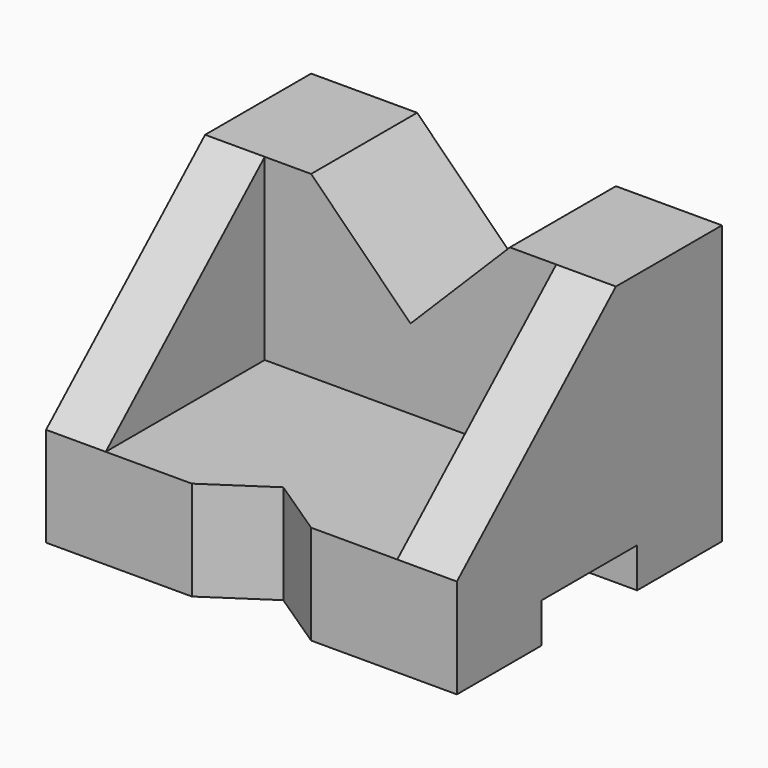
from build123d import *

# Parameters (mm, degrees)
F0_W      = 62
F0_H      = 15
F1_DEPTH  = 50
F3_DEPTH  = 20
F7_DEPTH  = 62
F8_DEPTH  = 9
F10_DEPTH = 25


# Not quite as in the source:
# - a pattern or mirror of a feature is missing from the dataset's text; its kind, count and spacing are read off the source's solid


with BuildPart() as f1:
    # F0 (on Front) → F1 (new body)
    with BuildSketch(Plane.XZ):
        with Locations((0, 7.5)):
            Rectangle(F0_W, F0_H)
    extrude(amount=F1_DEPTH)

    # F2 (on face) → F3 (join)
    with BuildSketch(Plane(origin=(0, 0, 0), x_dir=(-1, 0, 0), z_dir=(0, 1, 0))):
        Polygon((-31, 15), (31, 15), (31, 42), (15, 42), (0, 27), (-15, 42), (-31, 42), align=None)
    extrude(amount=-F3_DEPTH)

    # F5 (on face) → F7 (cut)
    with BuildSketch(Plane(origin=(-31, 0, 0), x_dir=(0, -1, 0), z_dir=(-1, 0, 0))):
        Polygon((16, 6), (16, 0), (25, 0), (34, 0), (34, 6), align=None)
    extrude(amount=-F7_DEPTH, mode=Mode.SUBTRACT)

    # F6 (on face) → F8 (join)
    with BuildSketch(Plane(origin=(-31, 0, 0), x_dir=(0, -1, 0), z_dir=(-1, 0, 0))):
        Polygon((50, 15), (20, 42), (20, 15), align=None)
    f8 = extrude(amount=-F8_DEPTH)

    # F8_copies: F8 across plane
    add(f8.mirror(Plane(origin=(0, 0, 0), x_dir=(0, 0, 1), z_dir=(1, 0, 0))))

    # F9 (on face) → F10 (cut)
    with BuildSketch(Plane.XY.offset(15)):
        Polygon((0, -44), (-9, -50), (9, -50), align=None)
    extrude(amount=-F10_DEPTH, mode=Mode.SUBTRACT)


solid = f1.part
